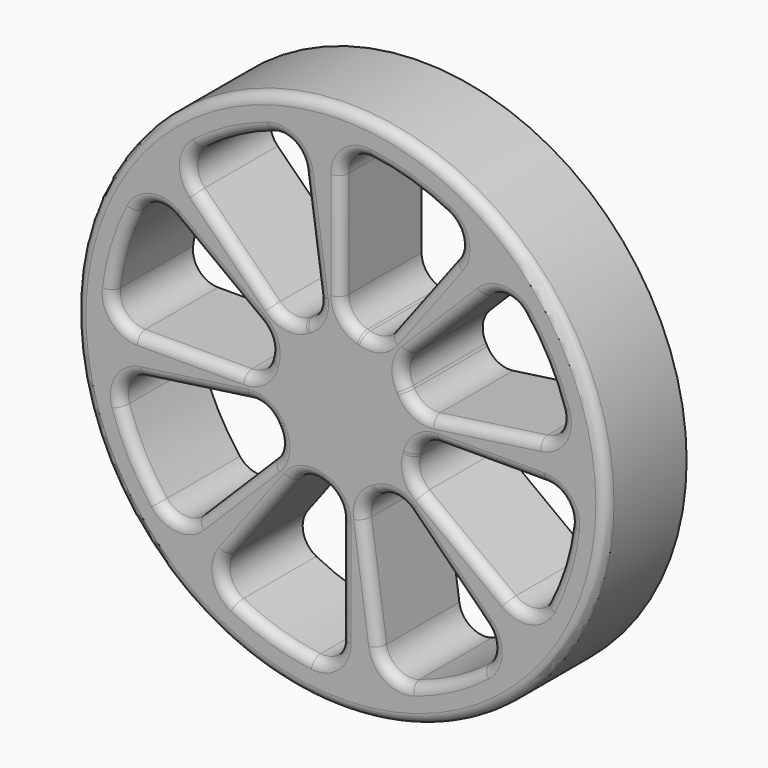
from build123d import *

# Parameters (mm, degrees)
F0_R            = 66.7448575271
F1_DEPTH        = 25.4
F3_DEPTH        = 25.4
F3_COPIES_COUNT = 8
F4_R            = 2.54


# Not quite as in the source:
# - a pattern or mirror of a feature is missing from the dataset's text; its kind, count and spacing are read off the source's solid


with BuildPart() as f1:
    # F0 (on Front) → F1 (new body)
    with BuildSketch(Plane.XZ):
        Circle(F0_R)
    extrude(amount=F1_DEPTH)

    # F2 (on face) → F3 (cut)
    with BuildSketch(Plane.XZ.offset(25.4)):
        with BuildLine():
            ThreePointArc((26.4919386824, 51.5813968349), (17.0739448109, 55.4160962463), (7.1308876249, 57.5466224575))
            ThreePointArc((7.1308876249, 57.5466224575), (2.1450110831, 56.0030305859), (0, 51.2448199759))
            Line((0, 51.2448199759), (0, 24.3969954913))
            ThreePointArc((0, 24.3969954913), (1.3260988677, 20.5133223057), (4.7505251694, 18.2517387623))
            ThreePointArc((4.7505251694, 18.2517387623), (5.0687699053, 18.1659304435), (5.3854664394, 18.0745735347))
            ThreePointArc((5.3854664394, 18.0745735347), (9.183779588, 18.1284264351), (12.2717067242, 20.340843419))
            Line((12.2717067242, 20.340843419), (28.6638498057, 42.1134966086))
            ThreePointArc((28.6638498057, 42.1134966086), (29.7801046894, 47.352627939), (26.4919386824, 51.5813968349))
        make_face()
    f3 = extrude(amount=-F3_DEPTH, mode=Mode.SUBTRACT)

    # F3_copies: F3 ×8 about axis
    f3_copies_axis = Axis((0, 0, 0), (0, 1, 0))
    for i in range(1, F3_COPIES_COUNT):
        add(f3.rotate(f3_copies_axis, i * 360 / F3_COPIES_COUNT), mode=Mode.SUBTRACT)

    # F4
    f4_edges = [f1.edges().sort_by_distance(p)[0] for p in [
        (-66.744858, -25.4, 0),
        (-20.467778, -25.4, -31.22717),
        (-9.18378, -25.4, -18.128426),
        (-29.780105, -25.4, -47.352628),
        (-5.06877, -25.4, -18.16593),
        (-17.073945, -25.4, -55.416096),
        (-1.326099, -25.4, -20.513322),
        (-2.145011, -25.4, -56.003031),
        (0, -25.4, -37.820908),
        (-36.553848, -25.4, -7.608039),
        (-19.312646, -25.4, -6.32482),
        (-54.541078, -25.4, -12.42565),
        (-16.429414, -25.4, -9.261091),
        (-51.2582, -25.4, -27.111995),
        (-15.442803, -25.4, -13.567416),
        (-41.116875, -25.4, -38.083371),
        (-26.74342, -25.4, -26.74342),
        (7.608039, -25.4, -36.553848),
        (6.32482, -25.4, -19.312646),
        (12.42565, -25.4, -54.541078),
        (9.261091, -25.4, -16.429414),
        (27.111995, -25.4, -51.2582),
        (13.567416, -25.4, -15.442803),
        (38.083371, -25.4, -41.116875),
        (26.74342, -25.4, -26.74342),
        (31.22717, -25.4, -20.467778),
        (18.128426, -25.4, -9.18378),
        (47.352628, -25.4, -29.780105),
        (18.16593, -25.4, -5.06877),
        (55.416096, -25.4, -17.073945),
        (20.513322, -25.4, -1.326099),
        (56.003031, -25.4, -2.145011),
        (37.820908, -25.4, 0),
        (-31.22717, -25.4, 20.467778),
        (-18.128426, -25.4, 9.18378),
        (-47.352628, -25.4, 29.780105),
        (-18.16593, -25.4, 5.06877),
        (-55.416096, -25.4, 17.073945),
        (-20.513322, -25.4, 1.326099),
        (-56.003031, -25.4, 2.145011),
        (-37.820908, -25.4, 0),
        (-7.608039, -25.4, 36.553848),
        (-12.42565, -25.4, 54.541078),
        (-27.111995, -25.4, 51.2582),
        (-38.083371, -25.4, 41.116875),
        (-26.74342, -25.4, 26.74342),
        (-13.567416, -25.4, 15.442803),
        (-9.261091, -25.4, 16.429414),
        (-6.32482, -25.4, 19.312646),
        (36.553848, -25.4, 7.608039),
        (19.312646, -25.4, 6.32482),
        (54.541078, -25.4, 12.42565),
        (16.429414, -25.4, 9.261091),
        (51.2582, -25.4, 27.111995),
        (15.442803, -25.4, 13.567416),
        (41.116875, -25.4, 38.083371),
        (26.74342, -25.4, 26.74342),
        (20.467778, -25.4, 31.22717),
        (9.18378, -25.4, 18.128426),
        (29.780105, -25.4, 47.352628),
        (5.06877, -25.4, 18.16593),
        (17.073945, -25.4, 55.416096),
        (1.326099, -25.4, 20.513322),
        (2.145011, -25.4, 56.003031),
        (0, -25.4, 37.820908),
    ]]
    fillet(f4_edges, radius=F4_R)


solid = f1.part
